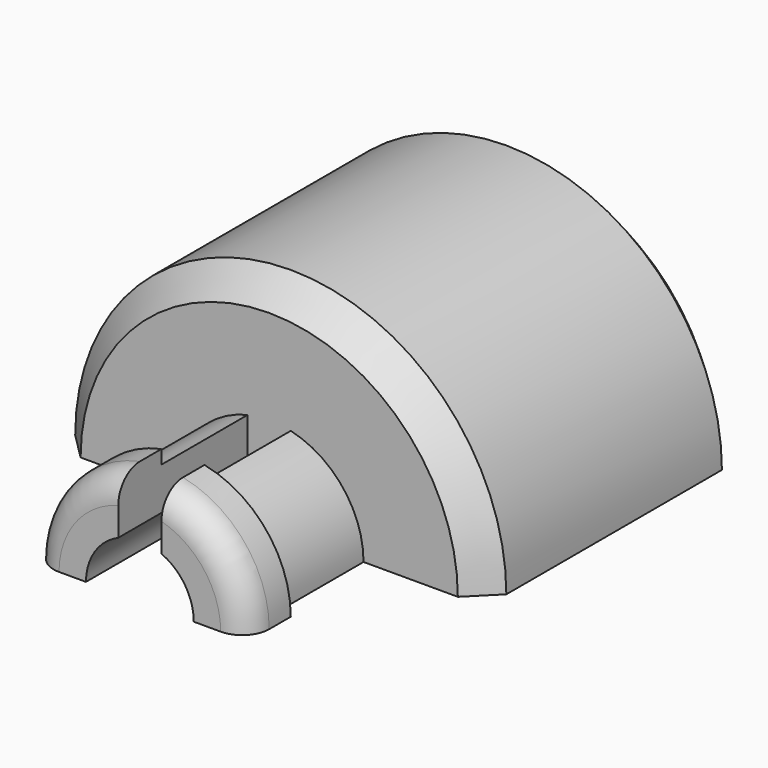
from build123d import *

# Parameters (mm, degrees)
F1_DEPTH = 6
F2_DEPTH = 3
F3_START = 2
F3_DEPTH = 1
F4_SIZE  = 0.5
F5_DEPTH = 8
F6_START = -7.5
F6_DEPTH = 0.5
F7_R     = 0.49999


# Not quite as in the source:
# - a fillet or chamfer is up to 0.001 mm smaller than in the source, because OpenCascade refuses the exact size


with BuildPart() as f1:
    # F0 (on Front) → F1 (new body)
    with BuildSketch(Plane.XZ):
        with BuildLine():
            Line((2, 0), (4, 0))
            ThreePointArc((4, 0), (0, 4), (-4, 0))
            Line((-4, 0), (-2, 0))
            ThreePointArc((-2, 0), (-1.5491933385, 1.2649110641), (-0.4, 1.9595917942))
            Line((-0.4, 1.9595917942), (-0.4, 2))
            Line((-0.4, 2), (0, 2))
            Line((0, 2), (0.4, 2))
            Line((0.4, 2), (0.4, 1.9595917942))
            ThreePointArc((0.4, 1.9595917942), (1.5491933385, 1.2649110641), (2, 0))
        make_face()
        with BuildLine():
            Line((1.75, 0), (2, 0))
            ThreePointArc((2, 0), (1.5491933385, 1.2649110641), (0.4, 1.9595917942))
            Line((0.4, 1.9595917942), (0.4, 1.7036725037))
            ThreePointArc((0.4, 1.7036725037), (1.3715866724, 1.086853256), (1.75, 0))
        make_face()
        with BuildLine():
            ThreePointArc((-0.4, 1.9595917942), (-1.5491933385, 1.2649110641), (-2, 0))
            Line((-2, 0), (-1.75, 0))
            ThreePointArc((-1.75, 0), (-1.3715866724, 1.086853256), (-0.4, 1.7036725037))
            Line((-0.4, 1.7036725037), (-0.4, 1.9595917942))
        make_face()
        with BuildLine():
            Line((1.2, 0), (1.75, 0))
            ThreePointArc((1.75, 0), (1.3715866724, 1.086853256), (0.4, 1.7036725037))
            Line((0.4, 1.7036725037), (0.4, 1.1313708499))
            ThreePointArc((0.4, 1.1313708499), (0.9797958971, 0.692820323), (1.2, 0))
        make_face()
        with BuildLine():
            ThreePointArc((0, 2), (0.201017924, 1.989872306), (0.4, 1.9595917942))
            Line((0.4, 1.9595917942), (0.4, 2))
            Line((0.4, 2), (0, 2))
        make_face()
        with BuildLine():
            Line((0.4, 1.7036725037), (0.4, 1.9595917942))
            ThreePointArc((0.4, 1.9595917942), (0.201017924, 1.989872306), (0, 2))
            ThreePointArc((0, 2), (-0.201017924, 1.989872306), (-0.4, 1.9595917942))
            Line((-0.4, 1.9595917942), (-0.4, 1.7036725037))
            ThreePointArc((-0.4, 1.7036725037), (0, 1.75), (0.4, 1.7036725037))
        make_face()
        with BuildLine():
            ThreePointArc((-0.4, 1.7036725037), (-1.3715866724, 1.086853256), (-1.75, 0))
            Line((-1.75, 0), (-1.2, 0))
            ThreePointArc((-1.2, 0), (-0.9797958971, 0.692820323), (-0.4, 1.1313708499))
            Line((-0.4, 1.1313708499), (-0.4, 1.7036725037))
        make_face()
        with BuildLine():
            Line((-0.4, 2), (-0.4, 1.9595917942))
            ThreePointArc((-0.4, 1.9595917942), (-0.201017924, 1.989872306), (0, 2))
            Line((0, 2), (-0.4, 2))
        make_face()
        with BuildLine():
            Line((1, 0), (1.2, 0))
            ThreePointArc((1.2, 0), (0.9797958971, 0.692820323), (0.4, 1.1313708499))
            Line((0.4, 1.1313708499), (0.4, 0.916515139))
            ThreePointArc((0.4, 0.916515139), (0.8366600265, 0.5477225575), (1, 0))
        make_face()
        with BuildLine():
            Line((0.4, 1.1313708499), (0.4, 1.7036725037))
            ThreePointArc((0.4, 1.7036725037), (0, 1.75), (-0.4, 1.7036725037))
            Line((-0.4, 1.7036725037), (-0.4, 1.1313708499))
            ThreePointArc((-0.4, 1.1313708499), (0, 1.2), (0.4, 1.1313708499))
        make_face()
        with BuildLine():
            ThreePointArc((-0.4, 1.1313708499), (-0.9797958971, 0.692820323), (-1.2, 0))
            Line((-1.2, 0), (-1, 0))
            ThreePointArc((-1, 0), (-0.8366600265, 0.5477225575), (-0.4, 0.916515139))
            Line((-0.4, 0.916515139), (-0.4, 1.1313708499))
        make_face()
        with BuildLine():
            Line((0.4, 0), (1, 0))
            ThreePointArc((1, 0), (0.8366600265, 0.5477225575), (0.4, 0.916515139))
            Line((0.4, 0.916515139), (0.4, 0))
        make_face()
        with BuildLine():
            Line((0.4, 0.916515139), (0.4, 1.1313708499))
            ThreePointArc((0.4, 1.1313708499), (0, 1.2), (-0.4, 1.1313708499))
            Line((-0.4, 1.1313708499), (-0.4, 0.916515139))
            ThreePointArc((-0.4, 0.916515139), (0, 1), (0.4, 0.916515139))
        make_face()
        with BuildLine():
            ThreePointArc((-0.4, 0.916515139), (-0.8366600265, 0.5477225575), (-1, 0))
            Line((-1, 0), (-0.4, 0))
            Line((-0.4, 0), (-0.4, 0.916515139))
        make_face()
        with BuildLine():
            Line((-0.4, 0), (0.4, 0))
            Line((0.4, 0), (0.4, 0.916515139))
            ThreePointArc((0.4, 0.916515139), (0, 1), (-0.4, 0.916515139))
            Line((-0.4, 0.916515139), (-0.4, 0))
        make_face()
    extrude(amount=-F1_DEPTH)

    # F0 (on Front) → F2 (join)
    with BuildSketch(Plane.XZ):
        with BuildLine():
            ThreePointArc((-0.4, 1.7036725037), (-1.3715866724, 1.086853256), (-1.75, 0))
            Line((-1.75, 0), (-1.2, 0))
            ThreePointArc((-1.2, 0), (-0.9797958971, 0.692820323), (-0.4, 1.1313708499))
            Line((-0.4, 1.1313708499), (-0.4, 1.7036725037))
        make_face()
        with BuildLine():
            Line((1, 0), (1.2, 0))
            ThreePointArc((1.2, 0), (0.9797958971, 0.692820323), (0.4, 1.1313708499))
            Line((0.4, 1.1313708499), (0.4, 0.916515139))
            ThreePointArc((0.4, 0.916515139), (0.8366600265, 0.5477225575), (1, 0))
        make_face()
        with BuildLine():
            Line((1.2, 0), (1.75, 0))
            ThreePointArc((1.75, 0), (1.3715866724, 1.086853256), (0.4, 1.7036725037))
            Line((0.4, 1.7036725037), (0.4, 1.1313708499))
            ThreePointArc((0.4, 1.1313708499), (0.9797958971, 0.692820323), (1.2, 0))
        make_face()
        with BuildLine():
            ThreePointArc((-0.4, 1.1313708499), (-0.9797958971, 0.692820323), (-1.2, 0))
            Line((-1.2, 0), (-1, 0))
            ThreePointArc((-1, 0), (-0.8366600265, 0.5477225575), (-0.4, 0.916515139))
            Line((-0.4, 0.916515139), (-0.4, 1.1313708499))
        make_face()
    extrude(amount=F2_DEPTH)

    # F0 (on Front) → F3 (join)
    with BuildSketch(Plane.XZ.offset(F3_START)):
        with BuildLine():
            Line((1.75, 0), (2, 0))
            ThreePointArc((2, 0), (1.5491933385, 1.2649110641), (0.4, 1.9595917942))
            Line((0.4, 1.9595917942), (0.4, 1.7036725037))
            ThreePointArc((0.4, 1.7036725037), (1.3715866724, 1.086853256), (1.75, 0))
        make_face()
        with BuildLine():
            ThreePointArc((-0.4, 1.9595917942), (-1.5491933385, 1.2649110641), (-2, 0))
            Line((-2, 0), (-1.75, 0))
            ThreePointArc((-1.75, 0), (-1.3715866724, 1.086853256), (-0.4, 1.7036725037))
            Line((-0.4, 1.7036725037), (-0.4, 1.9595917942))
        make_face()
    extrude(amount=F3_DEPTH)

    # F4
    f4_edges = [f1.edges().sort_by_distance(p)[0] for p in [
        (0, 0, 4),
        (0, 6, 4),
    ]]
    chamfer(f4_edges, length=F4_SIZE)

    # F0 (on Front) → F5 (join)
    with BuildSketch(Plane.XZ):
        with BuildLine():
            Line((0.4, 0), (1, 0))
            ThreePointArc((1, 0), (0.8366600265, 0.5477225575), (0.4, 0.916515139))
            Line((0.4, 0.916515139), (0.4, 0))
        make_face()
        with BuildLine():
            ThreePointArc((-0.4, 0.916515139), (-0.8366600265, 0.5477225575), (-1, 0))
            Line((-1, 0), (-0.4, 0))
            Line((-0.4, 0), (-0.4, 0.916515139))
        make_face()
    extrude(amount=-F5_DEPTH)

    # F0 (on Front) → F6 (join)
    with BuildSketch(Plane.XZ.offset(F6_START)):
        with BuildLine():
            ThreePointArc((-0.4, 1.1313708499), (-0.9797958971, 0.692820323), (-1.2, 0))
            Line((-1.2, 0), (-1, 0))
            ThreePointArc((-1, 0), (-0.8366600265, 0.5477225575), (-0.4, 0.916515139))
            Line((-0.4, 0.916515139), (-0.4, 1.1313708499))
        make_face()
        with BuildLine():
            Line((1, 0), (1.2, 0))
            ThreePointArc((1.2, 0), (0.9797958971, 0.692820323), (0.4, 1.1313708499))
            Line((0.4, 1.1313708499), (0.4, 0.916515139))
            ThreePointArc((0.4, 0.916515139), (0.8366600265, 0.5477225575), (1, 0))
        make_face()
    extrude(amount=-F6_DEPTH)

    # F7 (radius 0.5 in the source; OpenCascade refuses exactly that, so slightly less here)
    f7_edges = [f1.edges().sort_by_distance(p)[0] for p in [
        (0.979796, 8, 0.69282),
        (-0.979796, 8, 0.69282),
        (1.549193, -3, 1.264911),
        (-1.549193, -3, 1.264911),
    ]]
    fillet(f7_edges, radius=F7_R)


solid = f1.part
